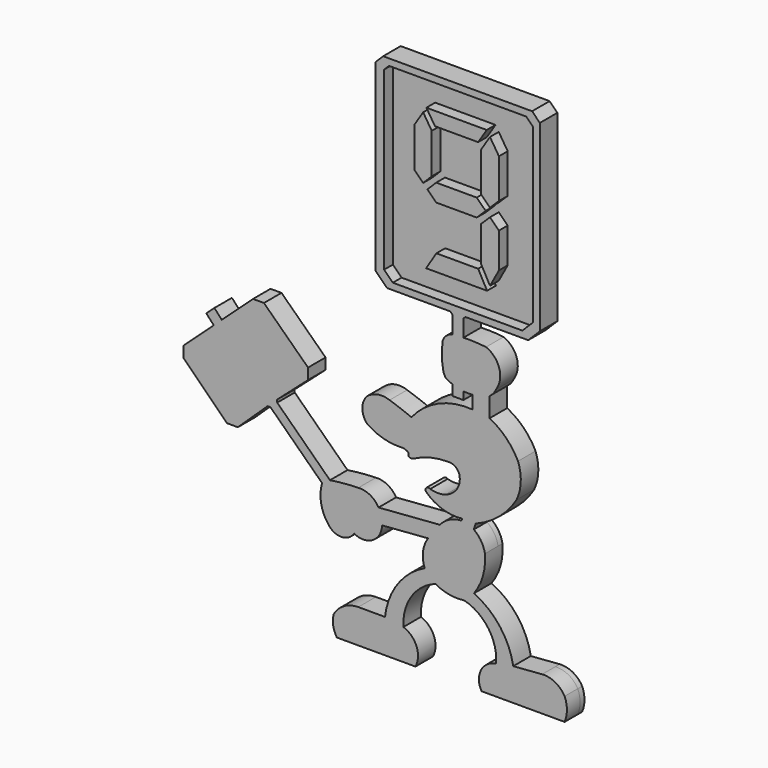
from build123d import *

# Parameters (mm, degrees)
F1_DEPTH = 3.81
F2_DEPTH = 1.27
F3_DEPTH = 1.27


with BuildPart() as f1:
    # F0 (on Front) → F1 (new body)
    with BuildSketch(Plane.XZ):
        with BuildLine():
            Line((-21.8629133387, 14.3691650665), (-24.4029133387, 14.3691650665))
            Line((-24.4029133387, 14.3691650665), (-31.6263630142, 7.750092945))
            Line((-31.6263630142, 7.750092945), (-33.3423621415, 9.6227773805))
            Line((-33.3423621415, 9.6227773805), (-35.215046577, 7.9067782531))
            Line((-35.215046577, 7.9067782531), (-33.4990474497, 6.0340938176))
            Line((-33.4990474497, 6.0340938176), (-40.483546324, -0.3660202358))
            Line((-40.483546324, -0.3660202358), (-40.483546324, -2.9060202358))
            Line((-40.483546324, -2.9060202358), (-30.4511819872, -12.9383845725))
            Line((-30.4511819872, -12.9383845725), (-27.9111819872, -12.9383845725))
            Line((-27.9111819872, -12.9383845725), (-21.0036390494, -6.3800711032))
            Line((-21.0036390494, -6.3800711032), (-20.3686390494, -6.3800711032))
            Line((-20.3686390494, -6.3800711032), (-8.3869188849, -17.9918755814))
            ThreePointArc((-8.3869188849, -17.9918755814), (-8.6271739068, -22.1824383427), (-6.8937429984, -26.0052326109))
            ThreePointArc((-6.8937429984, -26.0052326109), (-3.902701953, -27.5059766631), (-0.9836398046, -25.869628467))
            ThreePointArc((-0.9836398046, -25.869628467), (3.3146999245, -25.793437824), (5.4917495342, -22.0864195562))
            Line((5.4917495342, -22.0864195562), (16.1571671838, -21.2660491757))
            ThreePointArc((16.1571671838, -21.2660491757), (14.9876833405, -24.3421212605), (15.3586484172, -27.6120290333))
            ThreePointArc((15.3586484172, -27.6120290333), (9.1019902857, -32.8890303406), (6.1864759775, -40.5370555818))
            Line((6.1864759775, -40.5370555818), (0, -40.5370555818))
            ThreePointArc((0, -40.5370555818), (-3.2824129813, -41.412205893), (-5.6934449822, -43.8053309918))
            ThreePointArc((-5.6934449822, -43.8053309918), (-5.83669749, -46.1684983201), (-4.9671614542, -48.3705401421))
            Line((-4.9671614542, -48.3705401421), (13.2417995483, -48.3705401421))
            ThreePointArc((13.2417995483, -48.3705401421), (13.4812386772, -44.1492124062), (10.4404212907, -41.211463511))
            ThreePointArc((10.4404212907, -41.211463511), (12.2915106726, -34.3785455212), (17.8588870913, -30.0059467554))
            ThreePointArc((17.8588870913, -30.0059467554), (21.1080328406, -31.1462793155), (24.5510712266, -31.1991292983))
            ThreePointArc((24.5510712266, -31.1991292983), (30.1551239083, -35.1210974772), (31.9176577032, -41.7302362621))
            ThreePointArc((31.9176577032, -41.7302362621), (28.4196860912, -44.1633259868), (28.5456292331, -48.4224185348))
            Line((28.5456292331, -48.4224185348), (47.7921366692, -48.4224185348))
            ThreePointArc((47.7921366692, -48.4224185348), (48.3334002631, -45.8026118577), (47.7921366692, -43.1828051805))
            ThreePointArc((47.7921366692, -43.1828051805), (45.5893306206, -41.0391655235), (42.5810228679, -40.4085864785))
            Line((42.5810228679, -40.4085864785), (35.8928758981, -40.9176081973))
            ThreePointArc((35.8928758981, -40.9176081973), (32.8118360937, -33.848017294), (26.7990238365, -29.0191446951))
            ThreePointArc((26.7990238365, -29.0191446951), (28.8792533672, -24.7963299649), (29.3361085799, -20.1111616156))
            ThreePointArc((29.3361085799, -20.1111616156), (28.4480622977, -17.8101241527), (26.7526078969, -16.0188023001))
            Line((26.7526078969, -16.0188023001), (27.202744653, -14.6683941939))
            ThreePointArc((27.202744653, -14.6683941939), (32.6087069125, -11.4810813123), (36.6867855191, -6.7111058161))
            ThreePointArc((36.6867855191, -6.7111058161), (37.6383173334, -2.7597460062), (37.0000265539, 1.2541351607))
            ThreePointArc((37.0000265539, 1.2541351607), (34.2427731175, 5.0900610904), (30.4231904447, 7.8699104488))
            Line((30.4231904447, 7.8699104488), (30.4231904447, 12.4212158844))
            ThreePointArc((30.4231904447, 12.4212158844), (31.2858835204, 13.2208012874), (31.8972238287, 14.2257088389))
            ThreePointArc((31.8972238287, 14.2257088389), (32.6720073558, 18.733662059), (29.5848324895, 22.1087595529))
            ThreePointArc((29.5848324895, 22.1087595529), (26.9708194687, 22.32022546), (24.3482672113, 22.3189764914))
            Line((24.3482672113, 22.3189764914), (24.3482672113, 11.3995720702))
            ThreePointArc((24.3482672113, 11.3995720702), (25.4071227127, 11.3401047096), (26.466537267, 11.3886035979))
            Line((26.466537267, 11.3886035979), (26.466537267, 8.3516295999))
            ThreePointArc((26.466537267, 8.3516295999), (18.6222503626, 7.0248907492), (12.3157929629, 2.1749765147))
            ThreePointArc((12.3157929629, 2.1749765147), (9.7986425298, 3.1495369923), (7.2482923895, 4.0335780487))
            ThreePointArc((7.2482923895, 4.0335780487), (4.4930419392, 4.2732832751), (1.991830999, 3.0931106303))
            ThreePointArc((1.991830999, 3.0931106303), (0.9293330281, 0.3175208112), (1.991830999, -2.4580690078))
            ThreePointArc((1.991830999, -2.4580690078), (5.7224838336, -4.2356594493), (9.8259048536, -4.7250818461))
            ThreePointArc((9.8259048536, -4.7250818461), (10.764470219, -4.8158047454), (11.6031561047, -5.2467822097))
            ThreePointArc((11.6031561047, -5.2467822097), (11.6469135908, -5.6393938139), (11.6031561047, -6.0320054181))
            ThreePointArc((11.6031561047, -6.0320054181), (12.2405621757, -6.2162395954), (12.8838898901, -6.05388756))
            ThreePointArc((12.8838898901, -6.05388756), (16.7019931461, -4.6226047855), (20.7511578939, -4.1422427361))
            ThreePointArc((20.7511578939, -4.1422427361), (22.4290958599, -4.5597843117), (23.4312955284, -5.968831014))
            ThreePointArc((23.4312955284, -5.968831014), (23.3045958258, -8.081459019), (22.152367961, -9.8567395178))
            ThreePointArc((22.152367961, -9.8567395178), (21.2256067605, -10.5674095969), (20.1667100187, -11.0600311295))
            ThreePointArc((20.1667100187, -11.0600311295), (18.3983920146, -11.2932433564), (16.6300740105, -11.0600311295))
            ThreePointArc((16.6300740105, -11.0600311295), (15.7925123683, -11.038723658), (15.6372636571, -11.8620470152))
            ThreePointArc((15.6372636571, -11.8620470152), (19.5363319075, -14.2335543358), (24.0792048412, -14.6683941939))
            Line((24.0792048412, -14.6683941939), (23.9166137764, -15.1561666076))
            ThreePointArc((23.9166137764, -15.1561666076), (21.1399165741, -15.8326826081), (18.907905007, -17.617576335))
            Line((18.907905007, -17.617576335), (4.6847161412, -18.7116059591))
            ThreePointArc((4.6847161412, -18.7116059591), (2.7049782759, -16.7833635866), (0, -16.2171717559))
            ThreePointArc((0, -16.2171717559), (-3.2934229278, -16.401546833), (-6.5677667572, -16.8006724233))
            Line((-6.5677667572, -16.8006724233), (-18.7915849055, -4.954244334))
            Line((-18.7915849055, -4.954244334), (-18.7915849055, -4.319244334))
            Line((-18.7915849055, -4.319244334), (-11.6484221107, 1.9816167411))
            Line((-11.6484221107, 1.9816167411), (-11.6484221107, 4.5216167411))
            Line((-11.6484221107, 4.5216167411), (-21.8629133387, 14.3691650665))
        make_face()
        with BuildLine():
            ThreePointArc((21.7650010097, 12.0177058516), (23.0368516515, 11.6259653404), (24.3482672113, 11.3995720702))
            Line((24.3482672113, 11.3995720702), (24.3482672113, 22.3189764914))
            ThreePointArc((24.3482672113, 22.3189764914), (23.05452522, 22.2397832773), (21.7650010097, 22.1087595529))
            Line((21.7650010097, 22.1087595529), (21.7650010097, 12.0177058516))
        make_face()
        with BuildLine():
            ThreePointArc((20.3429460526, 12.6839792356), (21.0414003812, 12.3240071474), (21.7650010097, 12.0177058516))
            Line((21.7650010097, 12.0177058516), (21.7650010097, 22.1087595529))
            ThreePointArc((21.7650010097, 22.1087595529), (20.3960590322, 21.4349801326), (19.5563564351, 20.1610569036))
            ThreePointArc((19.5563564351, 20.1610569036), (19.3409533153, 17.1088163738), (19.6777544916, 14.0675771981))
            ThreePointArc((19.6777544916, 14.0675771981), (19.9329625839, 13.3385725845), (20.3429460526, 12.6839792356))
        make_face()
        with BuildLine():
            Line((24.3482672113, 9.5967361828), (24.3482672113, 11.3995720702))
            ThreePointArc((24.3482672113, 11.3995720702), (23.0368516515, 11.6259653404), (21.7650010097, 12.0177058516))
            Line((21.7650010097, 12.0177058516), (21.7650010097, 9.5967361828))
            Line((21.7650010097, 9.5967361828), (24.3482672113, 9.5967361828))
        make_face()
        with BuildLine():
            ThreePointArc((21.7650010097, 22.1087595529), (23.05452522, 22.2397832773), (24.3482672113, 22.3189764914))
            Line((24.3482672113, 22.3189764914), (24.3482672113, 26.2399246505))
            Line((24.3482672113, 26.2399246505), (24.7972800173, 26.6889374566))
            Line((24.7972800173, 26.6889374566), (39.360090181, 26.6889374566))
            Line((39.360090181, 26.6889374566), (42.0541670173, 29.3830142929))
            Line((42.0541670173, 29.3830142929), (42.0541670173, 71.8828862323))
            Line((42.0541670173, 71.8828862323), (40.2581157931, 73.6789374566))
            Line((40.2581157931, 73.6789374566), (5.7502182416, 73.6789374566))
            Line((5.7502182416, 73.6789374566), (3.9541670173, 71.8828862323))
            Line((3.9541670173, 71.8828862323), (3.9541670173, 29.3830142929))
            Line((3.9541670173, 29.3830142929), (6.6482438537, 26.6889374566))
            Line((6.6482438537, 26.6889374566), (21.3159882036, 26.6889374566))
            Line((21.3159882036, 26.6889374566), (21.7650010097, 26.2399246505))
            Line((21.7650010097, 26.2399246505), (21.7650010097, 22.1087595529))
        make_face()
        Polygon((7.0999002003, 72.1549374566), (38.9084338344, 72.1549374566), (40.4654107988, 70.5979604921), (40.4654107988, 30.6679400331), (38.0104082223, 28.2129374566), (7.9979258124, 28.2129374566), (5.9861670173, 30.2246962516), (5.9861670173, 71.0412042736), align=None, mode=Mode.SUBTRACT)
    extrude(amount=F1_DEPTH)



with BuildPart() as f1b:
    # F0 (on Front) → F1, piece 2 (new body)
    with BuildSketch(Plane.XZ):
        Polygon((29.8365958627, 33.6739374566), (27.7609715781, 37.4942682665), (18.0890447809, 37.4942682665), (15.710246876, 33.6739374566), align=None)
    extrude(amount=F1_DEPTH)


with BuildPart() as f1c:
    # F0 (on Front) → F1, piece 3 (new body)
    with BuildSketch(Plane.XZ):
        Polygon((32.5791468893, 46.8482052643), (28.4278983201, 46.8482052643), (28.4278983201, 38.7217933053), (30.5035226047, 34.9014624953), (32.5791468893, 38.7217933053), align=None)
        Polygon((32.5791468893, 46.8482052643), (30.5035226047, 48.8840988842), (28.4278983201, 46.8482052643), align=None)
    extrude(amount=F1_DEPTH)


with BuildPart() as f1d:
    # F0 (on Front) → F1, piece 4 (new body)
    with BuildSketch(Plane.XZ):
        Polygon((27.4305710702, 51.8982293653), (18.0460414534, 51.8982293653), (18.0460414534, 47.8264421255), (27.4305710702, 47.8264421255), (29.5061953548, 49.8623357454), align=None)
        Polygon((18.0460414534, 47.8264421255), (18.0460414534, 51.8982293653), (16.0101478335, 49.8623357454), align=None)
    extrude(amount=F1_DEPTH)


with BuildPart() as f1e:
    # F0 (on Front) → F1, piece 5 (new body)
    with BuildSketch(Plane.XZ):
        Polygon((17.0126756947, 52.8405199532), (17.0126750876, 62.1266552412), (13.0319636256, 62.1266552412), (13.0319636256, 52.8405199532), (15.0223196602, 50.8501639187), align=None)
        Polygon((17.0126750876, 62.1266552412), (15.0223193566, 65.2606593185), (13.0319636256, 62.1266552412), align=None)
    extrude(amount=F1_DEPTH)


with BuildPart() as f1f:
    # F0 (on Front) → F1, piece 6 (new body)
    with BuildSketch(Plane.XZ):
        Polygon((29.7545819708, 66.4399374566), (15.7712599906, 66.4399374566), (17.7616157216, 63.3059333793), (27.5936891326, 63.3059333793), (27.7642262398, 63.3059333793), align=None)
    extrude(amount=F1_DEPTH)


with BuildPart() as f1g:
    # F0 (on Front) → F1, piece 7 (new body)
    with BuildSketch(Plane.XZ):
        Polygon((32.5791468893, 61.9923918076), (30.5035226047, 65.2606593185), (28.4278983201, 61.9923918076), align=None)
        Polygon((32.5791468893, 61.9923918076), (28.4278983201, 61.9923918076), (28.4278983201, 52.8764662265), (30.5035226047, 50.8405726066), (32.5791468893, 52.8764662265), align=None)
    extrude(amount=F1_DEPTH)


with BuildPart() as f2:
    # F0 (on Front) → F2 (new body)
    with BuildSketch(Plane.XZ):
        Polygon((40.4654107988, 70.5979604921), (38.9084338344, 72.1549374566), (7.0999002003, 72.1549374566), (5.9861670173, 71.0412042736), (5.9861670173, 30.2246962516), (7.9979258124, 28.2129374566), (38.0104082223, 28.2129374566), (40.4654107988, 30.6679400331), align=None)
        Polygon((15.0223193566, 65.2606593185), (15.7712599906, 66.4399374566), (29.7545819708, 66.4399374566), (30.5035226047, 65.2606593185), (32.5791468893, 61.9923918076), (32.5791468893, 52.8764662265), (30.5035226047, 50.8405726066), (30.5035226047, 48.8840988842), (32.5791468893, 46.8482052643), (32.5791468893, 38.7217933053), (30.5035226047, 34.9014624953), (29.8365958627, 33.6739374566), (15.710246876, 33.6739374566), (18.0890447809, 37.4942682665), (27.7609715781, 37.4942682665), (28.4278983201, 38.7217933053), (28.4278983201, 46.8482052643), (27.4305710702, 47.8264421255), (18.0460414534, 47.8264421255), (16.0101478335, 49.8623357454), (15.0223196602, 50.8501639187), (13.0319636256, 52.8405199532), (13.0319636256, 62.1266552412), align=None, mode=Mode.SUBTRACT)
        Polygon((30.5035226047, 50.8405726066), (28.4278983201, 52.8764662265), (27.4305710702, 51.8982293653), (29.5061953548, 49.8623357454), align=None)
        Polygon((30.5035226047, 48.8840988842), (30.5035226047, 50.8405726066), (29.5061953548, 49.8623357454), align=None)
        Polygon((30.5035226047, 48.8840988842), (29.5061953548, 49.8623357454), (27.4305710702, 47.8264421255), (28.4278983201, 46.8482052643), align=None)
        Polygon((30.5035226047, 34.9014624953), (28.4278983201, 38.7217933053), (27.7609715781, 37.4942682665), (29.8365958627, 33.6739374566), align=None)
        Polygon((18.0460414534, 51.8982293653), (17.0126756947, 52.8405199532), (15.0223196602, 50.8501639187), (16.0101478335, 49.8623357454), align=None)
        Polygon((27.5936891326, 63.3059333793), (17.7616157216, 63.3059333793), (17.0126750876, 62.1266552412), (17.0126756947, 52.8405199532), (18.0460414534, 51.8982293653), (27.4305710702, 51.8982293653), (28.4278983201, 52.8764662265), (28.4278983201, 61.9923918076), align=None)
        Polygon((17.7616157216, 63.3059333793), (15.7712599906, 66.4399374566), (15.0223193566, 65.2606593185), (17.0126750876, 62.1266552412), align=None)
        Polygon((30.5035226047, 65.2606593185), (29.7545819708, 66.4399374566), (27.7642262398, 63.3059333793), (27.5936891326, 63.3059333793), (28.4278983201, 61.9923918076), align=None)
    extrude(amount=F2_DEPTH)


with BuildPart() as f1_1:
    add(f1.part)

    add(f1b.part)  # F3 merges F1b

    add(f1c.part)  # F3 merges F1c

    add(f1d.part)  # F3 merges F1d

    add(f1e.part)  # F3 merges F1e

    add(f1f.part)  # F3 merges F1f

    add(f1g.part)  # F3 merges F1g
    # F1_face (on face) + F2_face (on face) → F3 (join)
    with BuildSketch(Plane(origin=(30.5035226047, 0, 57.7656668441), x_dir=(1, 0, 0), z_dir=(0, 1, 0))):
        with BuildLine():
            ThreePointArc((-20.6776177511, 62.4907486902), (-24.7810387711, 62.0013262934), (-28.5116916057, 60.2237358519))
            ThreePointArc((-28.5116916057, 60.2237358519), (-29.5741895766, 57.4481460329), (-28.5116916057, 54.6725562138))
            ThreePointArc((-28.5116916057, 54.6725562138), (-26.0104806655, 53.492383569), (-23.2552302152, 53.7320887954))
            ThreePointArc((-23.2552302152, 53.7320887954), (-20.7048800749, 54.6161298518), (-18.1877296418, 55.5906903294))
            ThreePointArc((-18.1877296418, 55.5906903294), (-11.8812722421, 50.7407760949), (-4.0369853377, 49.4140372442))
            Line((-4.0369853377, 49.4140372442), (-4.0369853377, 46.3770632462))
            ThreePointArc((-4.0369853377, 46.3770632462), (-5.096399892, 46.4255621345), (-6.1552553934, 46.3660947739))
            Line((-6.1552553934, 46.3660947739), (-6.1552553934, 48.1689306613))
            Line((-6.1552553934, 48.1689306613), (-8.738521595, 48.1689306613))
            Line((-8.738521595, 48.1689306613), (-8.738521595, 45.7479609925))
            ThreePointArc((-8.738521595, 45.7479609925), (-9.4621222235, 45.4416596967), (-10.1605765522, 45.0816876085))
            ThreePointArc((-10.1605765522, 45.0816876085), (-10.5705600208, 44.4270942596), (-10.8257681131, 43.698089646))
            ThreePointArc((-10.8257681131, 43.698089646), (-11.1625692894, 40.6568504703), (-10.9471661696, 37.6046099405))
            ThreePointArc((-10.9471661696, 37.6046099405), (-10.1074635725, 36.3306867115), (-8.738521595, 35.6569072912))
            Line((-8.738521595, 35.6569072912), (-8.738521595, 31.5257421936))
            Line((-8.738521595, 31.5257421936), (-9.1875344011, 31.0767293875))
            Line((-9.1875344011, 31.0767293875), (-23.855278751, 31.0767293875))
            Line((-23.855278751, 31.0767293875), (-26.5493555874, 28.3826525512))
            Line((-26.5493555874, 28.3826525512), (-26.5493555874, -14.1172193882))
            Line((-26.5493555874, -14.1172193882), (-24.7533043631, -15.9132706125))
            Line((-24.7533043631, -15.9132706125), (9.7545931884, -15.9132706125))
            Line((9.7545931884, -15.9132706125), (11.5506444126, -14.1172193882))
            Line((11.5506444126, -14.1172193882), (11.5506444126, 28.3826525512))
            Line((11.5506444126, 28.3826525512), (8.8565675763, 31.0767293875))
            Line((8.8565675763, 31.0767293875), (-5.7062425874, 31.0767293875))
            Line((-5.7062425874, 31.0767293875), (-6.1552553934, 31.5257421936))
            Line((-6.1552553934, 31.5257421936), (-6.1552553934, 35.4466903527))
            ThreePointArc((-6.1552553934, 35.4466903527), (-3.532703136, 35.4454413841), (-0.9186901152, 35.6569072912))
            ThreePointArc((-0.9186901152, 35.6569072912), (2.1684847511, 39.0320047851), (1.393701224, 43.5399580052))
            ThreePointArc((1.393701224, 43.5399580052), (0.7823609157, 44.5448655567), (-0.08033216, 45.3444509597))
            Line((-0.08033216, 45.3444509597), (-0.08033216, 49.8957563953))
            ThreePointArc((-0.08033216, 49.8957563953), (3.7392505128, 52.6756057537), (6.4965039492, 56.5115316834))
            ThreePointArc((6.4965039492, 56.5115316834), (7.1347947287, 60.5254128503), (6.1832629144, 64.4767726602))
            ThreePointArc((6.1832629144, 64.4767726602), (2.1051843078, 69.2467481564), (-3.3007779517, 72.434061038))
            Line((-3.3007779517, 72.434061038), (-3.7509147078, 73.7844691442))
            ThreePointArc((-3.7509147078, 73.7844691442), (-2.055460307, 75.5757909969), (-1.1674140248, 77.8768284597))
            ThreePointArc((-1.1674140248, 77.8768284597), (-1.6242692375, 82.561996809), (-3.7044987682, 86.7848115392))
            ThreePointArc((-3.7044987682, 86.7848115392), (2.308313489, 91.6136841381), (5.3893532934, 98.6832750414))
            Line((5.3893532934, 98.6832750414), (12.0775002632, 98.1742533226))
            ThreePointArc((12.0775002632, 98.1742533226), (15.0858080159, 98.8048323676), (17.2886140645, 100.9484720247))
            ThreePointArc((17.2886140645, 100.9484720247), (17.8298776584, 103.5682787018), (17.2886140645, 106.1880853789))
            Line((17.2886140645, 106.1880853789), (-1.9578933716, 106.1880853789))
            ThreePointArc((-1.9578933716, 106.1880853789), (-2.0838365135, 101.9289928309), (1.4141350985, 99.4959031062))
            ThreePointArc((1.4141350985, 99.4959031062), (-0.3483986964, 92.8867643213), (-5.9524513781, 88.9647961424))
            ThreePointArc((-5.9524513781, 88.9647961424), (-9.3954897641, 88.9119461596), (-12.6446355134, 87.7716135995))
            ThreePointArc((-12.6446355134, 87.7716135995), (-18.2120119321, 92.1442123653), (-20.063101314, 98.9771303551))
            ThreePointArc((-20.063101314, 98.9771303551), (-17.0222839275, 101.9148792503), (-17.2617230564, 106.1362069862))
            Line((-17.2617230564, 106.1362069862), (-35.470684059, 106.1362069862))
            ThreePointArc((-35.470684059, 106.1362069862), (-36.3402200947, 103.9341651642), (-36.1969675869, 101.5709978359))
            ThreePointArc((-36.1969675869, 101.5709978359), (-33.785935586, 99.1778727371), (-30.5035226047, 98.3027224259))
            Line((-30.5035226047, 98.3027224259), (-24.3170466272, 98.3027224259))
            ThreePointArc((-24.3170466272, 98.3027224259), (-21.401532319, 90.6546971847), (-15.1448741875, 85.3776958774))
            ThreePointArc((-15.1448741875, 85.3776958774), (-15.5158392642, 82.1077881046), (-14.3463554209, 79.0317160198))
            Line((-14.3463554209, 79.0317160198), (-25.0117730705, 79.8520864003))
            ThreePointArc((-25.0117730705, 79.8520864003), (-27.1888226802, 83.5591046681), (-31.4871624093, 83.6352953111))
            ThreePointArc((-31.4871624093, 83.6352953111), (-34.4062245577, 85.2716435072), (-37.3972656031, 83.770899455))
            ThreePointArc((-37.3972656031, 83.770899455), (-39.1306965115, 79.9481051868), (-38.8904414896, 75.7575424255))
            Line((-38.8904414896, 75.7575424255), (-50.8721616541, 64.1457379473))
            Line((-50.8721616541, 64.1457379473), (-51.5071616541, 64.1457379473))
            Line((-51.5071616541, 64.1457379473), (-58.4147045919, 70.7040514166))
            Line((-58.4147045919, 70.7040514166), (-60.9547045919, 70.7040514166))
            Line((-60.9547045919, 70.7040514166), (-70.9870689287, 60.6716870799))
            Line((-70.9870689287, 60.6716870799), (-70.9870689287, 58.1316870799))
            Line((-70.9870689287, 58.1316870799), (-64.0025700544, 51.7315730265))
            Line((-64.0025700544, 51.7315730265), (-65.7185691817, 49.858888591))
            Line((-65.7185691817, 49.858888591), (-63.8458847462, 48.1428894636))
            Line((-63.8458847462, 48.1428894636), (-62.1298856189, 50.0155738991))
            Line((-62.1298856189, 50.0155738991), (-54.9064359434, 43.3965017776))
            Line((-54.9064359434, 43.3965017776), (-52.3664359434, 43.3965017776))
            Line((-52.3664359434, 43.3965017776), (-42.1519447154, 53.244050103))
            Line((-42.1519447154, 53.244050103), (-42.1519447154, 55.784050103))
            Line((-42.1519447154, 55.784050103), (-49.2951075102, 62.0849111781))
            Line((-49.2951075102, 62.0849111781), (-49.2951075102, 62.7199111781))
            Line((-49.2951075102, 62.7199111781), (-37.0712893619, 74.5663392674))
            ThreePointArc((-37.0712893619, 74.5663392674), (-33.7969455325, 74.1672136771), (-30.5035226047, 73.9828386))
            ThreePointArc((-30.5035226047, 73.9828386), (-27.7985443288, 74.5490304307), (-25.8188064635, 76.4772728032))
            Line((-25.8188064635, 76.4772728032), (-11.5956175977, 75.3832431791))
            ThreePointArc((-11.5956175977, 75.3832431791), (-9.3636060306, 73.5983494522), (-6.5869088283, 72.9218334517))
            Line((-6.5869088283, 72.9218334517), (-6.4243177635, 72.434061038))
            ThreePointArc((-6.4243177635, 72.434061038), (-10.9671906972, 71.9992211799), (-14.8662589476, 69.6277138593))
            ThreePointArc((-14.8662589476, 69.6277138593), (-14.7110102364, 68.8043905021), (-13.8734485942, 68.8256979736))
            ThreePointArc((-13.8734485942, 68.8256979736), (-12.1051305901, 69.0589102005), (-10.336812586, 68.8256979736))
            ThreePointArc((-10.336812586, 68.8256979736), (-9.2779158442, 68.333076441), (-8.3511546437, 67.6224063619))
            ThreePointArc((-8.3511546437, 67.6224063619), (-7.1989267789, 65.8471258631), (-7.0722270763, 63.7344978581))
            ThreePointArc((-7.0722270763, 63.7344978581), (-8.0744267448, 62.3254511558), (-9.7523647108, 61.9079095802))
            ThreePointArc((-9.7523647108, 61.9079095802), (-13.8015294586, 62.3882716296), (-17.6196327146, 63.8195544041))
            ThreePointArc((-17.6196327146, 63.8195544041), (-18.262960429, 63.9819064395), (-18.9003665, 63.7976722622))
            ThreePointArc((-18.9003665, 63.7976722622), (-18.8566090139, 63.405060658), (-18.9003665, 63.0124490538))
            ThreePointArc((-18.9003665, 63.0124490538), (-19.7390523857, 62.5814715895), (-20.6776177511, 62.4907486902))
        make_face()
        Polygon((-24.5173555874, -13.2755374295), (-24.5173555874, 27.5409705925), (-22.5055967923, 29.5527293875), (7.5068856176, 29.5527293875), (9.9618881941, 27.097726811), (9.9618881941, -12.832293648), (8.4049112297, -14.3892706125), (-23.4036224044, -14.3892706125), align=None, mode=Mode.SUBTRACT)
        Polygon((0, -7.4949924744), (2.0756242846, -4.2267249635), (2.0756242846, 4.8892006176), (0, 6.9250942375), (-2.0756242846, 4.8892006176), (-2.0756242846, -4.2267249635), align=None)
        Polygon((-13.49084691, 4.9251468909), (-15.4812029446, 6.9155029254), (-17.4715589791, 4.9251468909), (-17.4715589791, -4.3609883971), (-15.4812032481, -7.4949924744), (-13.4908475171, -4.3609883971), align=None)
        Polygon((-3.0729515345, 5.8674374788), (-0.9973272499, 7.9033310987), (-3.0729515345, 9.9392247186), (-12.4574811513, 9.9392247186), (-14.4933747712, 7.9033310987), (-12.4574811513, 5.8674374788), align=None)
        Polygon((-2.0756242846, 19.0438735388), (-2.0756242846, 10.9174615798), (0, 8.8815679599), (2.0756242846, 10.9174615798), (2.0756242846, 19.0438735388), (0, 22.8642043488), align=None)
        Polygon((-2.7425510266, 20.2713985776), (-0.666926742, 24.0917293875), (-14.7932757287, 24.0917293875), (-12.4144778238, 20.2713985776), align=None)
        Polygon((-14.7322626141, -8.6742706125), (-0.748940634, -8.6742706125), (-2.739296365, -5.5402665352), (-12.7419068831, -5.5402665352), align=None)
    with BuildSketch(Plane(origin=(23.0063260851, 0, 50.0455592926), x_dir=(1, 0, 0), z_dir=(0, 1, 0))):
        Polygon((17.4590847137, -20.5524011995), (17.4590847137, 19.3776192596), (15.0040821372, 21.8326218361), (-15.0084002727, 21.8326218361), (-17.0201590677, 19.820863041), (-17.0201590677, -20.995644981), (-15.9064258848, -22.1093781639), (15.9021077493, -22.1093781639), align=None)
        Polygon((-7.9840067284, -15.2151000259), (-9.9743624594, -12.0810959486), (-9.9743624594, -2.7949606606), (-7.9840064249, -0.8046046261), (-5.9936503904, -2.7949606606), (-5.9936509974, -12.0810959486), align=None, mode=Mode.SUBTRACT)
        Polygon((6.7482558857, -16.3943781639), (-7.2350660945, -16.3943781639), (-5.2447103635, -13.2603740866), (4.7579001547, -13.2603740866), align=None, mode=Mode.SUBTRACT)
        Polygon((9.5728208042, -11.946832515), (7.4971965196, -15.2151000259), (5.421572235, -11.946832515), (5.421572235, -2.8309069338), (7.4971965196, -0.7950133139), (9.5728208042, -2.8309069338), align=None, mode=Mode.SUBTRACT)
        Polygon((6.4998692697, 0.1832235472), (4.4242449851, -1.8526700727), (-4.9602846317, -1.8526700727), (-6.9961782516, 0.1832235472), (-4.9602846317, 2.2191171671), (4.4242449851, 2.2191171671), align=None, mode=Mode.SUBTRACT)
        Polygon((9.5728208042, 3.1973540283), (7.4971965196, 1.1614604084), (5.421572235, 3.1973540283), (5.421572235, 11.3237659873), (7.4971965196, 15.1440967973), (9.5728208042, 11.3237659873), align=None, mode=Mode.SUBTRACT)
        Polygon((-7.2960792091, 16.3716218361), (6.8302697776, 16.3716218361), (4.7546454931, 12.5512910261), (-4.9172813041, 12.5512910261), align=None, mode=Mode.SUBTRACT)
    extrude(amount=F3_DEPTH)


solid = Compound([f2.part, f1_1.part])
